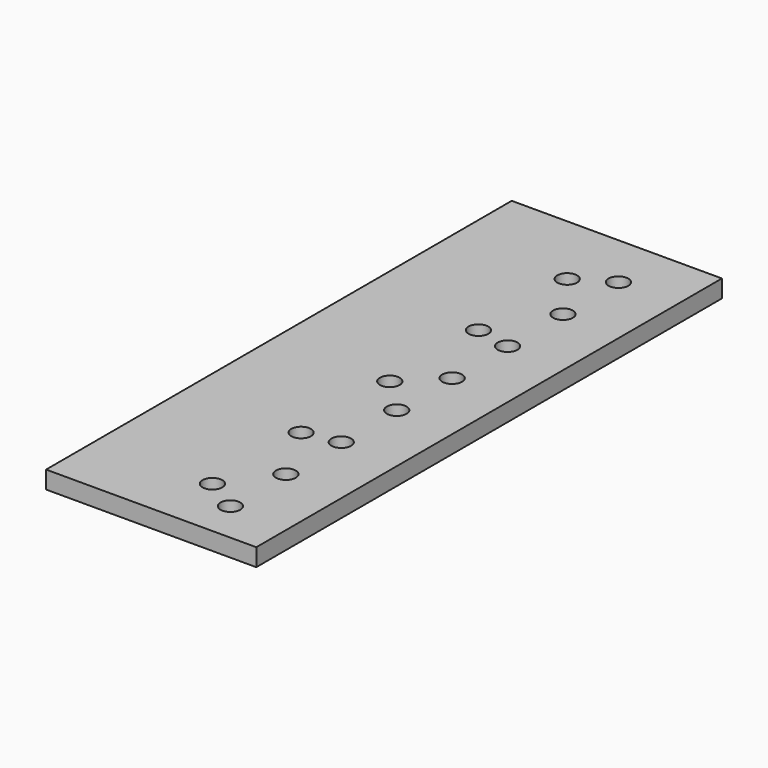
from build123d import *

# Parameters (mm, degrees)
F0_W           = 138.9888
F0_H           = 419.989
F1_DEPTH       = 12.7
F3_D           = 8.8
F3_CBORE_D     = 14.25
F3_CBORE_DEPTH = 8
F4_W           = 419.989
F4_H           = 12.7
F5_DEPTH       = 12.7


# Not quite as in the source:
# - a feature names something its author has since deleted; it is built from what else it names


with BuildPart() as f1:
    # F0 (on Top) → F1 (new body)
    with BuildSketch(Plane.XY):
        with Locations((69.4944, 309.9943)):
            Rectangle(F0_W, F0_H)
    extrude(amount=F1_DEPTH)

    # F3 (through all)
    with Locations(Plane.XY.offset(12.7)):
        with Locations((83.9978, 465.0339696), (83.9978, 385.0339772), (83.9978, 305.0339848), (83.9978, 225.0339924), (83.9978, 145.034), (108.9914, 130.0226), (108.9914, 180.0225), (108.9914, 230.0224), (108.9914, 280.0223), (108.9914, 330.0222), (108.9914, 380.0221), (108.9914, 430.022), (108.9914, 480.0219)):
            CounterBoreHole(F3_D / 2, F3_CBORE_D / 2, F3_CBORE_DEPTH)

    # F4 (on face) → F5 (join)
    with BuildSketch(Plane.YZ.offset(138.9888)):
        with Locations((309.9943, 6.35)):
            Rectangle(F4_W, F4_H)
    extrude(amount=F5_DEPTH)


solid = f1.part
